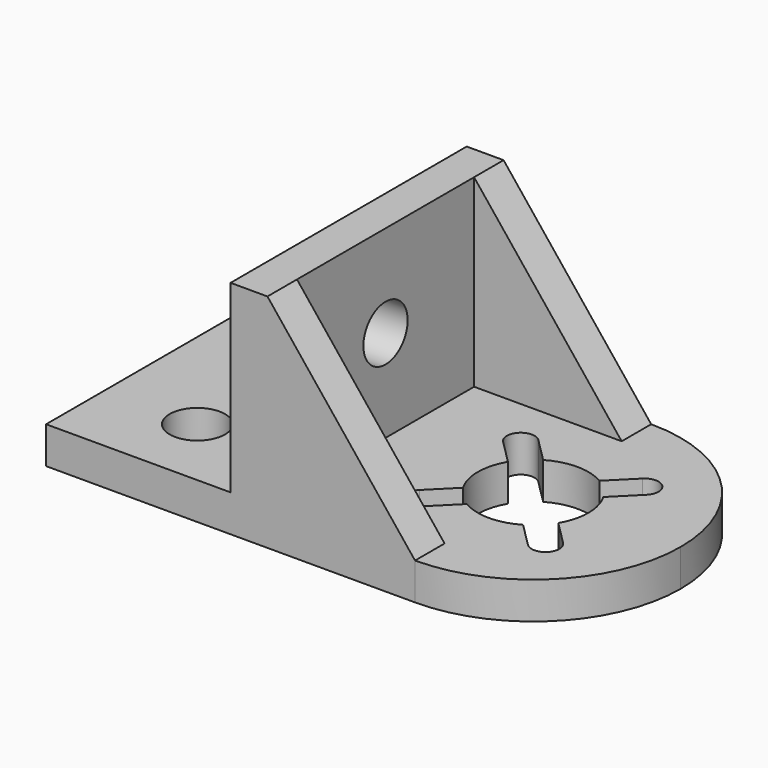
from build123d import *

# Parameters (mm, degrees)
F0_W     = 20
F0_H     = 32
F0_R     = 3
F1_DEPTH = 4
F2_DEPTH = 24
F3_W     = 16
F3_H     = 4
F4_DEPTH = 20
F5_SIZE2 = 19.99999
F5_SIZE  = 15.99999
F6_R     = 3
F7_DEPTH = 25


# Not quite as in the source:
# - a fillet or chamfer is up to 0.001 mm smaller than in the source, because OpenCascade refuses the exact size
# - a feature of the source that left no trace in its solid (it failed there, or was rolled back) is left out


with BuildPart() as f1:
    # F0 (on Top) → F1 (new body)
    with BuildSketch(Plane.XY):
        with BuildLine():
            ThreePointArc((20, 5), (31.313708499, 9.686291501), (36, 21))
            ThreePointArc((36, 21), (31.313708499, 32.313708499), (20, 37))
            ThreePointArc((20, 37), (8.686291501, 32.313708499), (4, 21))
            ThreePointArc((4, 21), (8.686291501, 9.686291501), (20, 5))
        make_face()
        with BuildLine():
            ThreePointArc((25.1685793531, 24.0472590095), (25.788414123, 22.5793232541), (26, 21))
            ThreePointArc((26, 21), (25.788414123, 19.4206767459), (25.1685793531, 17.9527409905))
            Line((25.1685793531, 17.9527409905), (27.7781745931, 15.3431457505))
            ThreePointArc((27.7781745931, 15.3431457505), (27.7781745931, 13.2218254069), (25.6568542495, 13.2218254069))
            Line((25.6568542495, 13.2218254069), (23.0472590095, 15.8314206469))
            ThreePointArc((23.0472590095, 15.8314206469), (20, 15), (16.9527409905, 15.8314206469))
            Line((16.9527409905, 15.8314206469), (14.3431457505, 13.2218254069))
            ThreePointArc((14.3431457505, 13.2218254069), (12.2218254069, 13.2218254069), (12.2218254069, 15.3431457505))
            Line((12.2218254069, 15.3431457505), (14.8314206469, 17.9527409905))
            ThreePointArc((14.8314206469, 17.9527409905), (14, 21), (14.8314206469, 24.0472590095))
            Line((14.8314206469, 24.0472590095), (12.2218254069, 26.6568542495))
            ThreePointArc((12.2218254069, 26.6568542495), (12.2218254069, 28.7781745931), (14.3431457505, 28.7781745931))
            Line((14.3431457505, 28.7781745931), (16.9527409905, 26.1685793531))
            ThreePointArc((16.9527409905, 26.1685793531), (20, 27), (23.0472590095, 26.1685793531))
            Line((23.0472590095, 26.1685793531), (25.6568542495, 28.7781745931))
            ThreePointArc((25.6568542495, 28.7781745931), (27.7781745931, 28.7781745931), (27.7781745931, 26.6568542495))
            Line((27.7781745931, 26.6568542495), (25.1685793531, 24.0472590095))
        make_face(mode=Mode.SUBTRACT)
        with BuildLine():
            ThreePointArc((4, 21), (8.686291501, 32.313708499), (20, 37))
            Line((20, 37), (4, 37))
            Line((4, 37), (4, 21))
        make_face()
        with BuildLine():
            Line((4, 5), (20, 5))
            ThreePointArc((20, 5), (8.686291501, 9.686291501), (4, 21))
            Line((4, 21), (4, 5))
        make_face()
        Polygon((4, 5), (4, 21), (4, 37), (0, 37), (0, 5), align=None)
        with Locations((-10, 21)):
            Rectangle(F0_W, F0_H)
        with Locations((-10, 13)):
            Circle(F0_R, mode=Mode.SUBTRACT)
        with Locations((-10, 29)):
            Circle(F0_R, mode=Mode.SUBTRACT)
    extrude(amount=F1_DEPTH)

    # F0 (on Top) → F2 (join)
    with BuildSketch(Plane.XY):
        Polygon((4, 5), (4, 21), (4, 37), (0, 37), (0, 5), align=None)
    extrude(amount=F2_DEPTH)

    # F3 (on face) → F4 (join)
    with BuildSketch(Plane.XY.offset(4)):
        with Locations((12, 7)):
            Rectangle(F3_W, F3_H)
        with Locations((12, 35)):
            Rectangle(F3_W, F3_H)
    extrude(amount=F4_DEPTH)

    # F5 (size 16 and 20 in the source; OpenCascade refuses exactly that, so slightly less here)
    f5_edges = [f1.edges().sort_by_distance(p)[0] for p in [
        (20, 7, 24),
        (20, 35, 24),
    ]]
    f5_side = f1.faces().sort_by_distance((3.622641, 21, 24))[0]
    chamfer(f5_edges, length=F5_SIZE, length2=F5_SIZE2, reference=f5_side)

    # F6 (on face) → F7 (cut)
    with BuildSketch(Plane.YZ.offset(4)):
        with Locations((21, 14)):
            Circle(F6_R)
    extrude(amount=-F7_DEPTH, mode=Mode.SUBTRACT)


solid = f1.part
